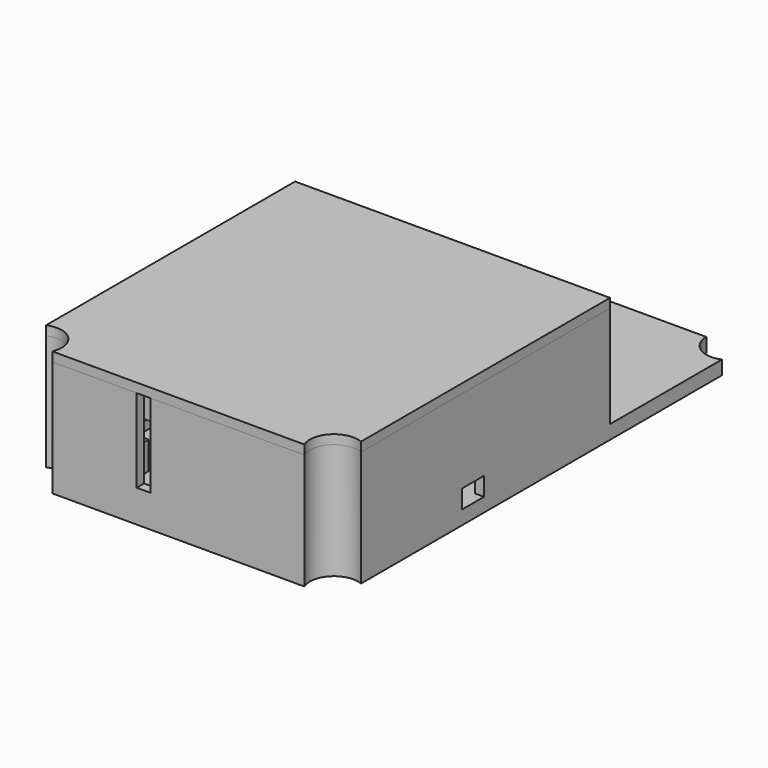
from build123d import *

# Parameters (mm, degrees)
F1_W      = 6
F1_H      = 12.5
F2_DEPTH  = 12.5
F4_DEPTH  = 11
F5_W      = 6
F5_H      = 6
F5_W_2    = 5
F6_DEPTH  = 3
F7_W      = 32
F7_H      = 1.8
F8_DEPTH  = 1
F10_DEPTH = 1
F12_DEPTH = 1
F13_W     = 1.5
F13_H     = 9
F14_DEPTH = 1
F15_W     = 34
F15_H     = 2
F16_DEPTH = 25
F17_DEPTH = 2
F18_SIZE  = 1.5
F19_W     = 9.7393654287
F19_H     = 17.2347798944
F20_DEPTH = 0.5
F21_W     = 3
F21_H     = 2
F22_DEPTH = 1


with BuildPart() as f2:
    # F1 (on Top) → F2 (new body)
    with BuildSketch(Plane.XY):
        with BuildLine():
            ThreePointArc((-13.4, 26.75), (-14.5577794898, 24.5866692347), (-17, 24.35))
            Line((-17, 24.35), (-17, -24.35))
            ThreePointArc((-17, -24.35), (-14.1615223689, -24.9115223689), (-13.6, -27.75))
            Line((-13.6, -27.75), (13.6, -27.75))
            ThreePointArc((13.6, -27.75), (14.1615223689, -24.9115223689), (17, -24.35))
            Line((17, -24.35), (17, 24.35))
            ThreePointArc((17, 24.35), (14.5577794898, 24.5866692347), (13.4, 26.75))
            Line((13.4, 26.75), (-13.4, 26.75))
        make_face()
        with Locations((-11, -13.5)):
            Rectangle(F1_W, F1_H, mode=Mode.SUBTRACT)
    extrude(amount=F2_DEPTH)

    # F3 (on face) → F4 (cut)
    with BuildSketch(Plane.XY.offset(12.5)):
        Polygon((-17, 9.25), (-16, 9.25), (-16, -22.5073593129), (-11.7573593129, -26.75), (11.7573593129, -26.75), (16, -22.5073593129), (16, 9.25), (17, 9.25), (17, 26.75), (-17, 26.75), align=None)
    extrude(amount=-F4_DEPTH, mode=Mode.SUBTRACT)

    # F5 (on face) → F6 (join)
    with BuildSketch(Plane.XY.offset(1.5)):
        with Locations((3, -24.75)):
            Rectangle(F5_W, F5_H)
        with Locations((-10.5, -24.75)):
            Rectangle(F5_W_2, F5_H)
    extrude(amount=F6_DEPTH)

    # F7 (on face) → F8 (join)
    with BuildSketch(Plane.XY.offset(1.5)):
        with Locations((0, 8.35)):
            Rectangle(F7_W, F7_H)
    extrude(amount=F8_DEPTH)

    # F13 (on face) → F14 (cut, through all)
    with BuildSketch(Plane.XZ.offset(27.75)):
        with Locations((-3.75, 8)):
            Rectangle(F13_W, F13_H)
    extrude(amount=-F14_DEPTH, mode=Mode.SUBTRACT)

    # F19 (on face) → F20 (join)
    with BuildSketch(Plane(origin=(0, 0, 0), x_dir=(1, 0, 0), z_dir=(0, 0, -1))):
        with Locations((-9.9391005933, 13.7184206396)):
            Rectangle(F19_W, F19_H)
    extrude(amount=-F20_DEPTH)

    # F21 (on face) → F22 (cut, through all)
    with BuildSketch(Plane(origin=(16, 0, 0), x_dir=(0, -1, 0), z_dir=(-1, 0, 0))):
        with Locations((9.25, 2.5)):
            Rectangle(F21_W, F21_H)
    extrude(amount=-F22_DEPTH, mode=Mode.SUBTRACT)


with BuildPart() as f10:
    # F9 (on face) → F10 (new body)
    with BuildSketch(Plane.XY.offset(12.5)):
        with BuildLine():
            Line((17, 9.25), (-17, 9.25))
            Line((-17, 9.25), (-17, -24.35))
            ThreePointArc((-17, -24.35), (-14.1615223689, -24.9115223689), (-13.6, -27.75))
            Line((-13.6, -27.75), (13.6, -27.75))
            ThreePointArc((13.6, -27.75), (14.1615223689, -24.9115223689), (17, -24.35))
            Line((17, -24.35), (17, 9.25))
        make_face()
    extrude(amount=F10_DEPTH)

    # F11 (on face) → F12 (join)
    with BuildSketch(Plane.XY.offset(12.5)):
        Polygon((15.8, 9.25), (-15.8, 9.25), (-15.8, -22.4245166004), (-11.6745166004, -26.55), (11.6745166004, -26.55), (15.8, -22.4245166004), align=None)
        Polygon((13.8, 7.45), (13.8, -21.5960894757), (10.8460894757, -24.55), (-10.8460894757, -24.55), (-13.8, -21.5960894757), (-13.8, 7.45), align=None, mode=Mode.SUBTRACT)
    extrude(amount=-F12_DEPTH)

    # F15 (on face) → F16 (cut)
    with BuildSketch(Plane(origin=(0, 0, 12.5), x_dir=(1, 0, 0), z_dir=(0, 0, -1))):
        with Locations((0, -6.45)):
            Rectangle(F15_W, F15_H)
    extrude(amount=F16_DEPTH, mode=Mode.SUBTRACT)

    # F17 (add): a face of the model
    f17_faces = [f10.faces().sort_by_distance(p)[0] for p in [
        (13.419252011, -24.169252011, 11.5),
    ]]
    extrude(f17_faces, amount=F17_DEPTH)

    # F18
    f18_edges = [f10.edges().sort_by_distance(p)[0] for p in [
        (-14.8, 5.45, 9.5),
        (14.8, 5.45, 9.5),
    ]]
    chamfer(f18_edges, length=F18_SIZE)


solid = Compound([f2.part, f10.part])
